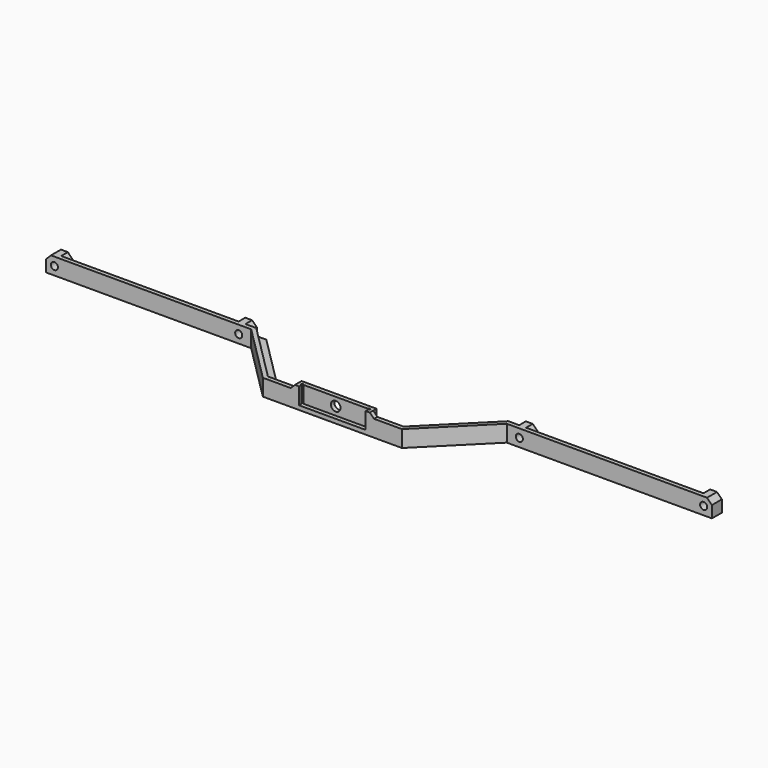
from build123d import *

# Parameters (mm, degrees)
F1_DEPTH  = 1.5875
F3_DEPTH  = 4.7625
F4_W      = 6.35
F4_H      = 6.35
F5_DEPTH  = 3.175
F6_SIZE   = 1.8598642
F7_W      = 28.575
F7_H      = 3.175
F8_DEPTH  = 1.5875
F9_W      = 25.4
F9_H      = 1.5875
F10_DEPTH = 6.35
F11_SIZE  = 1.58749
F12_R     = 1.35255
F12_R_2   = 1.8288
F13_DEPTH = 25.4
F14_R     = 0.396875
F15_DEPTH = 6.35


# Not quite as in the source:
# - a fillet or chamfer is up to 0.001 mm smaller than in the source, because OpenCascade refuses the exact size


with BuildPart() as f1:
    # F0 (on Top) → F1 (new body)
    with BuildSketch(Plane.XY):
        Polygon((-46.7826079092, 22.225), (-127, 22.225), (-127, 17.4625), (-48.7553, 17.4625), (-26.5303, -4.7625), (26.5303, -4.7625), (48.7553, 17.4625), (127, 17.4625), (127, 22.225), (46.7826079092, 22.225), (24.5576079092, 0), (-24.5576079092, 0), align=None)
    extrude(amount=F1_DEPTH)

    # F2 (on face) → F3 (join)
    with BuildSketch(Plane.XY.offset(1.5875)):
        Polygon((-127, 19.05), (-127, 17.4625), (-48.7553, 17.4625), (-26.5303, -4.7625), (26.5303, -4.7625), (48.7553, 17.4625), (127, 17.4625), (127, 19.05), (48.0977359697, 19.05), (25.8727359697, -3.175), (14.2875, -3.175), (14.2875, -1.5875), (-14.2875, -1.5875), (-14.2875, -3.175), (-25.8727359697, -3.175), (-48.0977359697, 19.05), align=None)
    extrude(amount=F3_DEPTH)

    # F4 (on face) → F5 (join, through all)
    with BuildSketch(Plane(origin=(0, 19.05, 0), x_dir=(-1, 0, 0), z_dir=(0, 1, 0))):
        with Locations((-53.5178, 3.175)):
            Rectangle(F4_W, F4_H)
        with Locations((-123.825, 3.175)):
            Rectangle(F4_W, F4_H)
        with Locations((123.825, 3.175)):
            Rectangle(F4_W, F4_H)
        with Locations((53.5178, 3.175)):
            Rectangle(F4_W, F4_H)
    extrude(amount=F5_DEPTH)

    # F6
    f6_edges = [f1.edges().sort_by_distance(p)[0] for p in [
        (-127, 19.84375, 6.35),
        (-120.65, 20.6375, 6.35),
        (-56.6928, 20.6375, 6.35),
        (-50.3428, 20.6375, 6.35),
        (50.3428, 20.6375, 6.35),
        (56.6928, 20.6375, 6.35),
        (120.65, 20.6375, 6.35),
        (127, 19.84375, 6.35),
    ]]
    chamfer(f6_edges, length=F6_SIZE)

    # F7 (on face) → F8 (join)
    with BuildSketch(Plane.XY.offset(6.35)):
        with Locations((0, -3.175)):
            Rectangle(F7_W, F7_H)
    extrude(amount=F8_DEPTH)

    # F9 (on face) → F10 (cut, through all)
    with BuildSketch(Plane.XY.offset(7.9375)):
        with Locations((0, -3.96875)):
            Rectangle(F9_W, F9_H)
    extrude(amount=-F10_DEPTH, mode=Mode.SUBTRACT)

    # F11 (size 1.5875 in the source; OpenCascade refuses exactly that, so slightly less here)
    f11_edges = [f1.edges().sort_by_distance(p)[0] for p in [
        (-14.2875, -3.96875, 6.35),
        (14.2875, -3.96875, 6.35),
    ]]
    chamfer(f11_edges, length=F11_SIZE)

    # F12 (on face) → F13 (cut, through all)
    with BuildSketch(Plane.XZ.offset(3.175)):
        with Locations((53.5178, 3.175)):
            Circle(F12_R)
        with Locations((123.825, 3.175)):
            Circle(F12_R)
        with Locations((-123.825, 3.175)):
            Circle(F12_R)
        with Locations((-53.5178, 3.175)):
            Circle(F12_R)
        with Locations((0, 4.7625)):
            Circle(F12_R_2)
    extrude(amount=-F13_DEPTH, mode=Mode.SUBTRACT)

    # F14 (on face) → F15 (cut, through all)
    with BuildSketch(Plane.XY.offset(7.9375)):
        with Locations((12.7, -3.175)):
            Circle(F14_R)
        with Locations((-12.7, -3.175)):
            Circle(F14_R)
    extrude(amount=-F15_DEPTH, mode=Mode.SUBTRACT)


solid = f1.part
